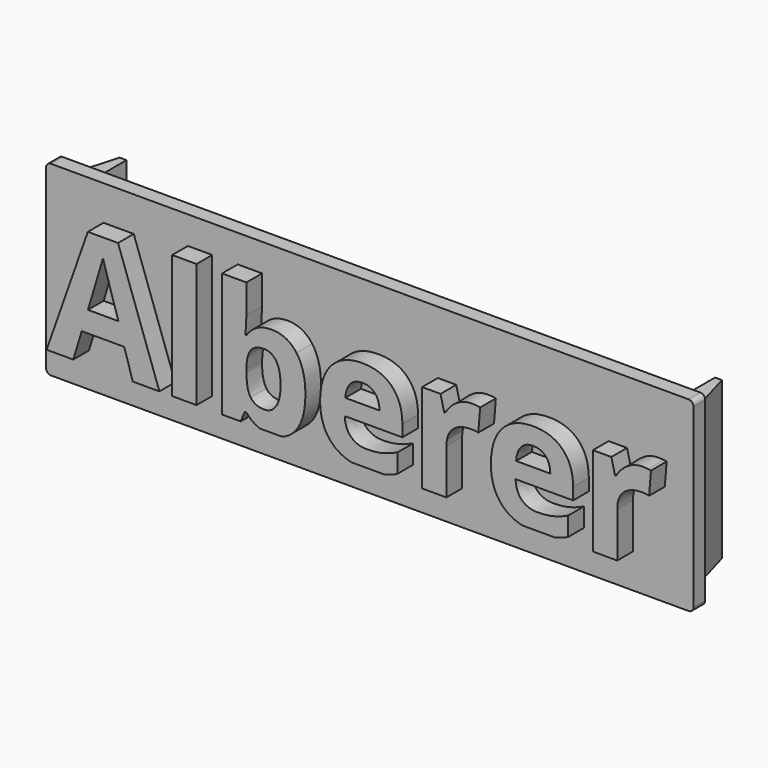
from build123d import *

# Parameters (mm, degrees)
F0_W     = 2.6041666667
F0_H     = 12
F0_W_2   = 2.4817708333
F0_W_3   = 1.2
F0_H_2   = 2
F0_H_3   = 1.5
F0_W_4   = 0.1463541667
F0_H_4   = 0.6640625
F0_W_5   = 0.5
F1_DEPTH = 1.5
F2_DEPTH = 3.5
F3_DEPTH = 5
F4_DEPTH = 1.5
F5_SIZE2 = 0.99999
F5_SIZE  = 3.49999
F6_SIZE2 = 3.49999
F6_SIZE  = 0.99999
F7_R     = 0.5


# Not quite as in the source:
# - a fillet or chamfer is up to 0.001 mm smaller than in the source, because OpenCascade refuses the exact size
# - a feature names something its author has since deleted; it is built from what else it names


with BuildPart() as f1:
    # F0 (on Front) → F1 (new body)
    with BuildSketch(Plane.XZ):
        with BuildLine():
            Line((30, 3.2387564007), (30, 6))
            Line((30, 6), (-10.9765625, 6))
            Line((-10.9765625, 6), (-10.9765625, 3.7161458333))
            add(Edge.make_bspline(
                [(-10.9765625, 3.7161458333), (-10.9765625, 3.15625), (-11.0729166667, 1.9192708333)],
                knots=[0, 0, 0, 1, 1, 1], degree=2))
            Line((-11.0729166667, 1.9192708333), (-10.9765625, 1.9192708333))
            add(Edge.make_bspline(
                [(-10.9765625, 1.9192708333), (-10.1041666667, 3.2682291667), (-8.3958333333, 3.2682291667)],
                knots=[0, 0, 0, 1, 1, 1], degree=2))
            add(Edge.make_bspline(
                [(-8.3958333333, 3.2682291667), (-6.7838541667, 3.2682291667), (-5.8723958333, 2.01171875)],
                knots=[0, 0, 0, 1, 1, 1], degree=2))
            add(Edge.make_bspline(
                [(-5.8723958333, 2.01171875), (-4.9609375, 0.7552083333), (-4.9609375, -1.4348958333)],
                knots=[0, 0, 0, 1, 1, 1], degree=2))
            add(Edge.make_bspline(
                [(-4.9609375, -1.4348958333), (-4.9609375, -3.6875), (-5.9010416667, -4.92578125)],
                knots=[0, 0, 0, 1, 1, 1], degree=2))
            add(Edge.make_bspline(
                [(-5.9010416667, -4.92578125), (-6.4989529355, -5.7133347356), (-7.3717996948, -6)],
                knots=[0, 0, 0, 0.6360053385, 0.6360053385, 0.6360053385], degree=2))
            Line((-7.3717996948, -6), (-0.2790829179, -6))
            add(Edge.make_bspline(
                [(-0.2790829179, -6), (-1.4444034881, -5.7178599903), (-2.2265625, -4.9505208333)],
                knots=[0.3676861883, 0.3676861883, 0.3676861883, 1, 1, 1], degree=2))
            add(Edge.make_bspline(
                [(-2.2265625, -4.9505208333), (-3.4635416667, -3.7369791667), (-3.4635416667, -1.515625)],
                knots=[0, 0, 0, 1, 1, 1], degree=2))
            add(Edge.make_bspline(
                [(-3.4635416667, -1.515625), (-3.4635416667, 0.7708333333), (-2.3203125, 2.01953125)],
                knots=[0, 0, 0, 1, 1, 1], degree=2))
            add(Edge.make_bspline(
                [(-2.3203125, 2.01953125), (-1.1770833333, 3.2682291667), (0.8411458333, 3.2682291667)],
                knots=[0, 0, 0, 1, 1, 1], degree=2))
            add(Edge.make_bspline(
                [(0.8411458333, 3.2682291667), (2.7682291667, 3.2682291667), (3.8424479167, 2.1705729167)],
                knots=[0, 0, 0, 1, 1, 1], degree=2))
            add(Edge.make_bspline(
                [(3.8424479167, 2.1705729167), (4.9166666667, 1.0729166667), (4.9166666667, -0.8645833333)],
                knots=[0, 0, 0, 1, 1, 1], degree=2))
            Line((4.9166666667, -0.8645833333), (4.9166666667, -2.0703125))
            Line((4.9166666667, -2.0703125), (-0.9505208333, -2.0703125))
            add(Edge.make_bspline(
                [(-0.9505208333, -2.0703125), (-0.9088541667, -3.1276041667), (-0.3229166667, -3.7213541667)],
                knots=[0, 0, 0, 1, 1, 1], degree=2))
            add(Edge.make_bspline(
                [(-0.3229166667, -3.7213541667), (0.2630208333, -4.3151041667), (1.3203125, -4.3151041667)],
                knots=[0, 0, 0, 1, 1, 1], degree=2))
            add(Edge.make_bspline(
                [(1.3203125, -4.3151041667), (2.1432291667, -4.3151041667), (2.875, -4.14453125)],
                knots=[0, 0, 0, 1, 1, 1], degree=2))
            add(Edge.make_bspline(
                [(2.875, -4.14453125), (3.6067708333, -3.9739583333), (4.4036458333, -3.5989583333)],
                knots=[0, 0, 0, 1, 1, 1], degree=2))
            Line((4.4036458333, -3.5989583333), (4.4036458333, -5.5208333333))
            add(Edge.make_bspline(
                [(4.4036458333, -5.5208333333), (3.7631867419, -5.841062879), (3.0370410498, -6)],
                knots=[0, 0, 0, 0.9837451644, 0.9837451644, 0.9837451644], degree=2))
            Line((3.0370410498, -6), (6.9348958333, -6))
            Line((6.9348958333, -6), (6.9348958333, 3.0989583333))
            Line((6.9348958333, 3.0989583333), (8.8151041667, 3.0989583333))
            Line((8.8151041667, 3.0989583333), (9.1822916667, 1.5677083333))
            Line((9.1822916667, 1.5677083333), (9.3020833333, 1.5677083333))
            add(Edge.make_bspline(
                [(9.3020833333, 1.5677083333), (9.7265625, 2.3333333333), (10.4466145833, 2.80078125)],
                knots=[0, 0, 0, 1, 1, 1], degree=2))
            add(Edge.make_bspline(
                [(10.4466145833, 2.80078125), (11.1666666667, 3.2682291667), (12.0130208333, 3.2682291667)],
                knots=[0, 0, 0, 1, 1, 1], degree=2))
            add(Edge.make_bspline(
                [(12.0130208333, 3.2682291667), (12.5182291667, 3.2682291667), (12.8515625, 3.1953125)],
                knots=[0, 0, 0, 1, 1, 1], degree=2))
            Line((12.8515625, 3.1953125), (12.6640625, 0.8697916667))
            add(Edge.make_bspline(
                [(12.6640625, 0.8697916667), (12.3619791667, 0.9505208333), (11.9322916667, 0.9505208333)],
                knots=[0, 0, 0, 1, 1, 1], degree=2))
            add(Edge.make_bspline(
                [(11.9322916667, 0.9505208333), (10.7447916667, 0.9505208333), (10.0807291667, 0.33984375)],
                knots=[0, 0, 0, 1, 1, 1], degree=2))
            add(Edge.make_bspline(
                [(10.0807291667, 0.33984375), (9.4166666667, -0.2708333333), (9.4166666667, -1.3697916667)],
                knots=[0, 0, 0, 1, 1, 1], degree=2))
            Line((9.4166666667, -1.3697916667), (9.4166666667, -6))
            Line((9.4166666667, -6), (17.1349795821, -6))
            add(Edge.make_bspline(
                [(17.1349795821, -6), (15.9696590119, -5.7178599903), (15.1875, -4.9505208333)],
                knots=[0.3676861883, 0.3676861883, 0.3676861883, 1, 1, 1], degree=2))
            add(Edge.make_bspline(
                [(15.1875, -4.9505208333), (13.9505208333, -3.7369791667), (13.9505208333, -1.515625)],
                knots=[0, 0, 0, 1, 1, 1], degree=2))
            add(Edge.make_bspline(
                [(13.9505208333, -1.515625), (13.9505208333, 0.7708333333), (15.09375, 2.01953125)],
                knots=[0, 0, 0, 1, 1, 1], degree=2))
            add(Edge.make_bspline(
                [(15.09375, 2.01953125), (16.2369791667, 3.2682291667), (18.2552083333, 3.2682291667)],
                knots=[0, 0, 0, 1, 1, 1], degree=2))
            add(Edge.make_bspline(
                [(18.2552083333, 3.2682291667), (20.1822916667, 3.2682291667), (21.2565104167, 2.1705729167)],
                knots=[0, 0, 0, 1, 1, 1], degree=2))
            add(Edge.make_bspline(
                [(21.2565104167, 2.1705729167), (22.3307291667, 1.0729166667), (22.3307291667, -0.8645833333)],
                knots=[0, 0, 0, 1, 1, 1], degree=2))
            Line((22.3307291667, -0.8645833333), (22.3307291667, -2.0703125))
            Line((22.3307291667, -2.0703125), (16.4635416667, -2.0703125))
            add(Edge.make_bspline(
                [(16.4635416667, -2.0703125), (16.5052083333, -3.1276041667), (17.0911458333, -3.7213541667)],
                knots=[0, 0, 0, 1, 1, 1], degree=2))
            add(Edge.make_bspline(
                [(17.0911458333, -3.7213541667), (17.6770833333, -4.3151041667), (18.734375, -4.3151041667)],
                knots=[0, 0, 0, 1, 1, 1], degree=2))
            add(Edge.make_bspline(
                [(18.734375, -4.3151041667), (19.5572916667, -4.3151041667), (20.2890625, -4.14453125)],
                knots=[0, 0, 0, 1, 1, 1], degree=2))
            add(Edge.make_bspline(
                [(20.2890625, -4.14453125), (21.0208333333, -3.9739583333), (21.8177083333, -3.5989583333)],
                knots=[0, 0, 0, 1, 1, 1], degree=2))
            Line((21.8177083333, -3.5989583333), (21.8177083333, -5.5208333333))
            add(Edge.make_bspline(
                [(21.8177083333, -5.5208333333), (21.1772492419, -5.841062879), (20.4511035498, -6)],
                knots=[0, 0, 0, 0.9837451644, 0.9837451644, 0.9837451644], degree=2))
            Line((20.4511035498, -6), (24.3489583333, -6))
            Line((24.3489583333, -6), (24.3489583333, 3.0989583333))
            Line((24.3489583333, 3.0989583333), (26.2291666667, 3.0989583333))
            Line((26.2291666667, 3.0989583333), (26.5963541667, 1.5677083333))
            Line((26.5963541667, 1.5677083333), (26.7161458333, 1.5677083333))
            add(Edge.make_bspline(
                [(26.7161458333, 1.5677083333), (27.140625, 2.3333333333), (27.8606770833, 2.80078125)],
                knots=[0, 0, 0, 1, 1, 1], degree=2))
            add(Edge.make_bspline(
                [(27.8606770833, 2.80078125), (28.5807291667, 3.2682291667), (29.4270833333, 3.2682291667)],
                knots=[0, 0, 0, 1, 1, 1], degree=2))
            add(Edge.make_bspline(
                [(29.4270833333, 3.2682291667), (29.7482774266, 3.2682291667), (30, 3.2387564007)],
                knots=[0, 0, 0, 0.6357656279, 0.6357656279, 0.6357656279], degree=2))
        make_face()
        with BuildLine():
            Line((-30, -9.5), (30, -9.5))
            Line((30, -9.5), (30, -8))
            Line((30, -8), (30, -6))
            Line((30, -6), (26.8307291667, -6))
            Line((26.8307291667, -6), (24.3489583333, -6))
            Line((24.3489583333, -6), (20.4511035498, -6))
            add(Edge.make_bspline(
                [(20.4511035498, -6), (20.4391051388, -6.002626185), (20.4270833333, -6.0052083333)],
                knots=[0.9837451644, 0.9837451644, 0.9837451644, 1, 1, 1], degree=2))
            add(Edge.make_bspline(
                [(20.4270833333, -6.0052083333), (19.6875, -6.1640625), (18.6197916667, -6.1640625)],
                knots=[0, 0, 0, 1, 1, 1], degree=2))
            add(Edge.make_bspline(
                [(18.6197916667, -6.1640625), (17.8126055815, -6.1640625), (17.1349795821, -6)],
                knots=[0, 0, 0, 0.3676861883, 0.3676861883, 0.3676861883], degree=2))
            Line((17.1349795821, -6), (9.4166666667, -6))
            Line((9.4166666667, -6), (6.9348958333, -6))
            Line((6.9348958333, -6), (3.0370410498, -6))
            add(Edge.make_bspline(
                [(3.0370410498, -6), (3.0250426388, -6.002626185), (3.0130208333, -6.0052083333)],
                knots=[0.9837451644, 0.9837451644, 0.9837451644, 1, 1, 1], degree=2))
            add(Edge.make_bspline(
                [(3.0130208333, -6.0052083333), (2.2734375, -6.1640625), (1.2057291667, -6.1640625)],
                knots=[0, 0, 0, 1, 1, 1], degree=2))
            add(Edge.make_bspline(
                [(1.2057291667, -6.1640625), (0.3985430815, -6.1640625), (-0.2790829179, -6)],
                knots=[0, 0, 0, 0.3676861883, 0.3676861883, 0.3676861883], degree=2))
            Line((-0.2790829179, -6), (-7.3717996948, -6))
            add(Edge.make_bspline(
                [(-7.3717996948, -6), (-7.8713419807, -6.1640625), (-8.4609375, -6.1640625)],
                knots=[0.6360053385, 0.6360053385, 0.6360053385, 1, 1, 1], degree=2))
            add(Edge.make_bspline(
                [(-8.4609375, -6.1640625), (-9.0631725128, -6.1640625), (-9.567777492, -6)],
                knots=[0, 0, 0, 0.3754192288, 0.3754192288, 0.3754192288], degree=2))
            Line((-9.567777492, -6), (-11.5625, -6))
            Line((-11.5625, -6), (-13.4583333333, -6))
            Line((-13.4583333333, -6), (-16.0625, -6))
            Line((-16.0625, -6), (-18.5442708333, -6))
            Line((-18.5442708333, -6), (-19.8463541667, -6))
            Line((-19.8463541667, -6), (-22.5651041667, -6))
            Line((-22.5651041667, -6), (-28.6276041667, -6))
            Line((-28.6276041667, -6), (-30, -6))
            Line((-30, -6), (-30, -8))
            Line((-30, -8), (-30, -9.5))
        make_face()
        Polygon((30, 8), (30, 9.5), (-30, 9.5), (-30, 8), (-30, 6), (-18.5442708333, 6), (-18.5442708333, 6.6640625), (-16.0625, 6.6640625), (-16.0625, 6), (-13.4583333333, 6), (-13.4583333333, 6.6640625), (-10.9765625, 6.6640625), (-10.9765625, 6), (30, 6), align=None)
        with BuildLine():
            Line((-10.9765625, 3.7161458333), (-10.9765625, 6))
            Line((-10.9765625, 6), (-13.4583333333, 6))
            Line((-13.4583333333, 6), (-13.4583333333, -6))
            Line((-13.4583333333, -6), (-11.5625, -6))
            Line((-11.5625, -6), (-11.1458333333, -5))
            Line((-11.1458333333, -5), (-10.9765625, -5))
            add(Edge.make_bspline(
                [(-9.567777492, -6), (-10.4072831512, -5.727051054), (-10.9765625, -5)],
                knots=[0.3754192288, 0.3754192288, 0.3754192288, 1, 1, 1], degree=2))
            Line((-9.567777492, -6), (-7.3717996948, -6))
            add(Edge.make_bspline(
                [(-5.9010416667, -4.92578125), (-6.4989529355, -5.7133347356), (-7.3717996948, -6)],
                knots=[0, 0, 0, 0.6360053385, 0.6360053385, 0.6360053385], degree=2))
            add(Edge.make_bspline(
                [(-4.9609375, -1.4348958333), (-4.9609375, -3.6875), (-5.9010416667, -4.92578125)],
                knots=[0, 0, 0, 1, 1, 1], degree=2))
            add(Edge.make_bspline(
                [(-5.8723958333, 2.01171875), (-4.9609375, 0.7552083333), (-4.9609375, -1.4348958333)],
                knots=[0, 0, 0, 1, 1, 1], degree=2))
            add(Edge.make_bspline(
                [(-8.3958333333, 3.2682291667), (-6.7838541667, 3.2682291667), (-5.8723958333, 2.01171875)],
                knots=[0, 0, 0, 1, 1, 1], degree=2))
            add(Edge.make_bspline(
                [(-10.9765625, 1.9192708333), (-10.1041666667, 3.2682291667), (-8.3958333333, 3.2682291667)],
                knots=[0, 0, 0, 1, 1, 1], degree=2))
            Line((-10.9765625, 1.9192708333), (-11.0729166667, 1.9192708333))
            add(Edge.make_bspline(
                [(-10.9765625, 3.7161458333), (-10.9765625, 3.15625), (-11.0729166667, 1.9192708333)],
                knots=[0, 0, 0, 1, 1, 1], degree=2))
        make_face()
        with BuildLine():
            add(Edge.make_bspline(
                [(-9.1927083333, 1.2838541667), (-10.1145833333, 1.2838541667), (-10.5377604167, 0.71875)],
                knots=[0, 0, 0, 1, 1, 1], degree=2))
            add(Edge.make_bspline(
                [(-7.9479166667, 0.6119791667), (-8.4036458333, 1.2838541667), (-9.1927083333, 1.2838541667)],
                knots=[0, 0, 0, 1, 1, 1], degree=2))
            add(Edge.make_bspline(
                [(-7.4921875, -1.4010416667), (-7.4921875, -0.0598958333), (-7.9479166667, 0.6119791667)],
                knots=[0, 0, 0, 1, 1, 1], degree=2))
            add(Edge.make_bspline(
                [(-7.9440104167, -3.44921875), (-7.4921875, -2.7447916667), (-7.4921875, -1.4010416667)],
                knots=[0, 0, 0, 1, 1, 1], degree=2))
            add(Edge.make_bspline(
                [(-9.1614583333, -4.1536458333), (-8.3958333333, -4.1536458333), (-7.9440104167, -3.44921875)],
                knots=[0, 0, 0, 1, 1, 1], degree=2))
            add(Edge.make_bspline(
                [(-10.5403645833, -3.5182291667), (-10.1041666667, -4.1536458333), (-9.1614583333, -4.1536458333)],
                knots=[0, 0, 0, 1, 1, 1], degree=2))
            add(Edge.make_bspline(
                [(-10.9765625, -1.4192708333), (-10.9765625, -2.8828125), (-10.5403645833, -3.5182291667)],
                knots=[0, 0, 0, 1, 1, 1], degree=2))
            Line((-10.9765625, -1.4192708333), (-10.9765625, -1.1484375))
            add(Edge.make_bspline(
                [(-10.5377604167, 0.71875), (-10.9609375, 0.1536458333), (-10.9765625, -1.1484375)],
                knots=[0, 0, 0, 1, 1, 1], degree=2))
        make_face(mode=Mode.SUBTRACT)
        Polygon((-30, -2.170444565), (-30, -6), (-28.6276041667, -6), (-27.765625, -3.1666666667), (-23.4270833333, -3.1666666667), (-22.5651041667, -6), (-19.8463541667, -6), (-24.0625, 5.9479166667), (-27.1458333333, 5.9479166667), align=None)
        with BuildLine():
            add(Edge.make_bspline(
                [(-24.03125, -1.0520833333), (-25.2265625, 2.796875), (-25.3776041667, 3.3020833333)],
                knots=[0, 0, 0, 1, 1, 1], degree=2))
            Line((-24.03125, -1.0520833333), (-27.1302083333, -1.0520833333))
            add(Edge.make_bspline(
                [(-25.59375, 4.0989583333), (-25.8619791667, 3.0572916667), (-27.1302083333, -1.0520833333)],
                knots=[0, 0, 0, 1, 1, 1], degree=2))
            add(Edge.make_bspline(
                [(-25.3776041667, 3.3020833333), (-25.5286458333, 3.8072916667), (-25.59375, 4.0989583333)],
                knots=[0, 0, 0, 1, 1, 1], degree=2))
        make_face(mode=Mode.SUBTRACT)
        with BuildLine():
            Line((-0.2790829179, -6), (3.0370410498, -6))
            add(Edge.make_bspline(
                [(4.4036458333, -5.5208333333), (3.7631867419, -5.841062879), (3.0370410498, -6)],
                knots=[0, 0, 0, 0.9837451644, 0.9837451644, 0.9837451644], degree=2))
            Line((4.4036458333, -5.5208333333), (4.4036458333, -3.5989583333))
            add(Edge.make_bspline(
                [(2.875, -4.14453125), (3.6067708333, -3.9739583333), (4.4036458333, -3.5989583333)],
                knots=[0, 0, 0, 1, 1, 1], degree=2))
            add(Edge.make_bspline(
                [(1.3203125, -4.3151041667), (2.1432291667, -4.3151041667), (2.875, -4.14453125)],
                knots=[0, 0, 0, 1, 1, 1], degree=2))
            add(Edge.make_bspline(
                [(-0.3229166667, -3.7213541667), (0.2630208333, -4.3151041667), (1.3203125, -4.3151041667)],
                knots=[0, 0, 0, 1, 1, 1], degree=2))
            add(Edge.make_bspline(
                [(-0.9505208333, -2.0703125), (-0.9088541667, -3.1276041667), (-0.3229166667, -3.7213541667)],
                knots=[0, 0, 0, 1, 1, 1], degree=2))
            Line((-0.9505208333, -2.0703125), (4.9166666667, -2.0703125))
            Line((4.9166666667, -2.0703125), (4.9166666667, -0.8645833333))
            add(Edge.make_bspline(
                [(3.8424479167, 2.1705729167), (4.9166666667, 1.0729166667), (4.9166666667, -0.8645833333)],
                knots=[0, 0, 0, 1, 1, 1], degree=2))
            add(Edge.make_bspline(
                [(0.8411458333, 3.2682291667), (2.7682291667, 3.2682291667), (3.8424479167, 2.1705729167)],
                knots=[0, 0, 0, 1, 1, 1], degree=2))
            add(Edge.make_bspline(
                [(-2.3203125, 2.01953125), (-1.1770833333, 3.2682291667), (0.8411458333, 3.2682291667)],
                knots=[0, 0, 0, 1, 1, 1], degree=2))
            add(Edge.make_bspline(
                [(-3.4635416667, -1.515625), (-3.4635416667, 0.7708333333), (-2.3203125, 2.01953125)],
                knots=[0, 0, 0, 1, 1, 1], degree=2))
            add(Edge.make_bspline(
                [(-2.2265625, -4.9505208333), (-3.4635416667, -3.7369791667), (-3.4635416667, -1.515625)],
                knots=[0, 0, 0, 1, 1, 1], degree=2))
            add(Edge.make_bspline(
                [(-0.2790829179, -6), (-1.4444034881, -5.7178599903), (-2.2265625, -4.9505208333)],
                knots=[0.3676861883, 0.3676861883, 0.3676861883, 1, 1, 1], degree=2))
        make_face()
        with BuildLine():
            add(Edge.make_bspline(
                [(0.8567708333, 1.5026041667), (0.0677083333, 1.5026041667), (-0.3802083333, 1.0026041667)],
                knots=[0, 0, 0, 1, 1, 1], degree=2))
            add(Edge.make_bspline(
                [(2.109375, 1.0026041667), (1.6458333333, 1.5026041667), (0.8567708333, 1.5026041667)],
                knots=[0, 0, 0, 1, 1, 1], degree=2))
            add(Edge.make_bspline(
                [(2.5911458333, -0.4166666667), (2.5729166667, 0.5026041667), (2.109375, 1.0026041667)],
                knots=[0, 0, 0, 1, 1, 1], degree=2))
            Line((2.5911458333, -0.4166666667), (-0.8932291667, -0.4166666667))
            add(Edge.make_bspline(
                [(-0.3802083333, 1.0026041667), (-0.828125, 0.5026041667), (-0.8932291667, -0.4166666667)],
                knots=[0, 0, 0, 1, 1, 1], degree=2))
        make_face(mode=Mode.SUBTRACT)
        with BuildLine():
            Line((17.1349795821, -6), (20.4511035498, -6))
            add(Edge.make_bspline(
                [(21.8177083333, -5.5208333333), (21.1772492419, -5.841062879), (20.4511035498, -6)],
                knots=[0, 0, 0, 0.9837451644, 0.9837451644, 0.9837451644], degree=2))
            Line((21.8177083333, -5.5208333333), (21.8177083333, -3.5989583333))
            add(Edge.make_bspline(
                [(20.2890625, -4.14453125), (21.0208333333, -3.9739583333), (21.8177083333, -3.5989583333)],
                knots=[0, 0, 0, 1, 1, 1], degree=2))
            add(Edge.make_bspline(
                [(18.734375, -4.3151041667), (19.5572916667, -4.3151041667), (20.2890625, -4.14453125)],
                knots=[0, 0, 0, 1, 1, 1], degree=2))
            add(Edge.make_bspline(
                [(17.0911458333, -3.7213541667), (17.6770833333, -4.3151041667), (18.734375, -4.3151041667)],
                knots=[0, 0, 0, 1, 1, 1], degree=2))
            add(Edge.make_bspline(
                [(16.4635416667, -2.0703125), (16.5052083333, -3.1276041667), (17.0911458333, -3.7213541667)],
                knots=[0, 0, 0, 1, 1, 1], degree=2))
            Line((16.4635416667, -2.0703125), (22.3307291667, -2.0703125))
            Line((22.3307291667, -2.0703125), (22.3307291667, -0.8645833333))
            add(Edge.make_bspline(
                [(21.2565104167, 2.1705729167), (22.3307291667, 1.0729166667), (22.3307291667, -0.8645833333)],
                knots=[0, 0, 0, 1, 1, 1], degree=2))
            add(Edge.make_bspline(
                [(18.2552083333, 3.2682291667), (20.1822916667, 3.2682291667), (21.2565104167, 2.1705729167)],
                knots=[0, 0, 0, 1, 1, 1], degree=2))
            add(Edge.make_bspline(
                [(15.09375, 2.01953125), (16.2369791667, 3.2682291667), (18.2552083333, 3.2682291667)],
                knots=[0, 0, 0, 1, 1, 1], degree=2))
            add(Edge.make_bspline(
                [(13.9505208333, -1.515625), (13.9505208333, 0.7708333333), (15.09375, 2.01953125)],
                knots=[0, 0, 0, 1, 1, 1], degree=2))
            add(Edge.make_bspline(
                [(15.1875, -4.9505208333), (13.9505208333, -3.7369791667), (13.9505208333, -1.515625)],
                knots=[0, 0, 0, 1, 1, 1], degree=2))
            add(Edge.make_bspline(
                [(17.1349795821, -6), (15.9696590119, -5.7178599903), (15.1875, -4.9505208333)],
                knots=[0.3676861883, 0.3676861883, 0.3676861883, 1, 1, 1], degree=2))
        make_face()
        with BuildLine():
            add(Edge.make_bspline(
                [(18.2708333333, 1.5026041667), (17.4817708333, 1.5026041667), (17.0338541667, 1.0026041667)],
                knots=[0, 0, 0, 1, 1, 1], degree=2))
            add(Edge.make_bspline(
                [(19.5234375, 1.0026041667), (19.0598958333, 1.5026041667), (18.2708333333, 1.5026041667)],
                knots=[0, 0, 0, 1, 1, 1], degree=2))
            add(Edge.make_bspline(
                [(20.0052083333, -0.4166666667), (19.9869791667, 0.5026041667), (19.5234375, 1.0026041667)],
                knots=[0, 0, 0, 1, 1, 1], degree=2))
            Line((20.0052083333, -0.4166666667), (16.5208333333, -0.4166666667))
            add(Edge.make_bspline(
                [(17.0338541667, 1.0026041667), (16.5859375, 0.5026041667), (16.5208333333, -0.4166666667)],
                knots=[0, 0, 0, 1, 1, 1], degree=2))
        make_face(mode=Mode.SUBTRACT)
        Polygon((-30, 6), (-30, -2.170444565), (-27.1458333333, 5.9479166667), (-24.0625, 5.9479166667), (-19.8463541667, -6), (-18.5442708333, -6), (-18.5442708333, 6), align=None)
        with Locations((-14.7604166667, 0)):
            Rectangle(F0_W, F0_H)
        with Locations((-17.3033854167, 0)):
            Rectangle(F0_W_2, F0_H)
        with BuildLine():
            Line((6.9348958333, -6), (9.4166666667, -6))
            Line((9.4166666667, -6), (9.4166666667, -1.3697916667))
            add(Edge.make_bspline(
                [(10.0807291667, 0.33984375), (9.4166666667, -0.2708333333), (9.4166666667, -1.3697916667)],
                knots=[0, 0, 0, 1, 1, 1], degree=2))
            add(Edge.make_bspline(
                [(11.9322916667, 0.9505208333), (10.7447916667, 0.9505208333), (10.0807291667, 0.33984375)],
                knots=[0, 0, 0, 1, 1, 1], degree=2))
            add(Edge.make_bspline(
                [(12.6640625, 0.8697916667), (12.3619791667, 0.9505208333), (11.9322916667, 0.9505208333)],
                knots=[0, 0, 0, 1, 1, 1], degree=2))
            Line((12.6640625, 0.8697916667), (12.8515625, 3.1953125))
            add(Edge.make_bspline(
                [(12.0130208333, 3.2682291667), (12.5182291667, 3.2682291667), (12.8515625, 3.1953125)],
                knots=[0, 0, 0, 1, 1, 1], degree=2))
            add(Edge.make_bspline(
                [(10.4466145833, 2.80078125), (11.1666666667, 3.2682291667), (12.0130208333, 3.2682291667)],
                knots=[0, 0, 0, 1, 1, 1], degree=2))
            add(Edge.make_bspline(
                [(9.3020833333, 1.5677083333), (9.7265625, 2.3333333333), (10.4466145833, 2.80078125)],
                knots=[0, 0, 0, 1, 1, 1], degree=2))
            Line((9.3020833333, 1.5677083333), (9.1822916667, 1.5677083333))
            Line((9.1822916667, 1.5677083333), (8.8151041667, 3.0989583333))
            Line((8.8151041667, 3.0989583333), (6.9348958333, 3.0989583333))
            Line((6.9348958333, 3.0989583333), (6.9348958333, -6))
        make_face()
        with BuildLine():
            Line((24.3489583333, -6), (26.8307291667, -6))
            Line((26.8307291667, -6), (26.8307291667, -1.3697916667))
            add(Edge.make_bspline(
                [(27.4947916667, 0.33984375), (26.8307291667, -0.2708333333), (26.8307291667, -1.3697916667)],
                knots=[0, 0, 0, 1, 1, 1], degree=2))
            add(Edge.make_bspline(
                [(29.3463541667, 0.9505208333), (28.1588541667, 0.9505208333), (27.4947916667, 0.33984375)],
                knots=[0, 0, 0, 1, 1, 1], degree=2))
            add(Edge.make_bspline(
                [(30, 0.888848029), (29.7219184932, 0.9505208333), (29.3463541667, 0.9505208333)],
                knots=[0.1259593855, 0.1259593855, 0.1259593855, 1, 1, 1], degree=2))
            Line((30, 0.888848029), (30, 3.2387564007))
            add(Edge.make_bspline(
                [(29.4270833333, 3.2682291667), (29.7482774266, 3.2682291667), (30, 3.2387564007)],
                knots=[0, 0, 0, 0.6357656279, 0.6357656279, 0.6357656279], degree=2))
            add(Edge.make_bspline(
                [(27.8606770833, 2.80078125), (28.5807291667, 3.2682291667), (29.4270833333, 3.2682291667)],
                knots=[0, 0, 0, 1, 1, 1], degree=2))
            add(Edge.make_bspline(
                [(26.7161458333, 1.5677083333), (27.140625, 2.3333333333), (27.8606770833, 2.80078125)],
                knots=[0, 0, 0, 1, 1, 1], degree=2))
            Line((26.7161458333, 1.5677083333), (26.5963541667, 1.5677083333))
            Line((26.5963541667, 1.5677083333), (26.2291666667, 3.0989583333))
            Line((26.2291666667, 3.0989583333), (24.3489583333, 3.0989583333))
            Line((24.3489583333, 3.0989583333), (24.3489583333, -6))
        make_face()
        Polygon((31.7, -9.5), (33, -9.5), (33, 9.5), (31.7, 9.5), (31.7, 8), (31.7, -8), align=None)
        Polygon((-33, -9.5), (-31.7, -9.5), (-31.7, -8), (-31.7, 8), (-31.7, 9.5), (-33, 9.5), align=None)
        with BuildLine():
            Line((26.8307291667, -6), (30, -6))
            Line((30, -6), (30, 0.888848029))
            add(Edge.make_bspline(
                [(30, 0.888848029), (29.7219184932, 0.9505208333), (29.3463541667, 0.9505208333)],
                knots=[0.1259593855, 0.1259593855, 0.1259593855, 1, 1, 1], degree=2))
            add(Edge.make_bspline(
                [(29.3463541667, 0.9505208333), (28.1588541667, 0.9505208333), (27.4947916667, 0.33984375)],
                knots=[0, 0, 0, 1, 1, 1], degree=2))
            add(Edge.make_bspline(
                [(27.4947916667, 0.33984375), (26.8307291667, -0.2708333333), (26.8307291667, -1.3697916667)],
                knots=[0, 0, 0, 1, 1, 1], degree=2))
            Line((26.8307291667, -1.3697916667), (26.8307291667, -6))
        make_face()
        with BuildLine():
            add(Edge.make_bspline(
                [(-7.9479166667, 0.6119791667), (-8.4036458333, 1.2838541667), (-9.1927083333, 1.2838541667)],
                knots=[0, 0, 0, 1, 1, 1], degree=2))
            add(Edge.make_bspline(
                [(-9.1927083333, 1.2838541667), (-10.1145833333, 1.2838541667), (-10.5377604167, 0.71875)],
                knots=[0, 0, 0, 1, 1, 1], degree=2))
            add(Edge.make_bspline(
                [(-10.5377604167, 0.71875), (-10.9609375, 0.1536458333), (-10.9765625, -1.1484375)],
                knots=[0, 0, 0, 1, 1, 1], degree=2))
            Line((-10.9765625, -1.1484375), (-10.9765625, -1.4192708333))
            add(Edge.make_bspline(
                [(-10.9765625, -1.4192708333), (-10.9765625, -2.8828125), (-10.5403645833, -3.5182291667)],
                knots=[0, 0, 0, 1, 1, 1], degree=2))
            add(Edge.make_bspline(
                [(-10.5403645833, -3.5182291667), (-10.1041666667, -4.1536458333), (-9.1614583333, -4.1536458333)],
                knots=[0, 0, 0, 1, 1, 1], degree=2))
            add(Edge.make_bspline(
                [(-9.1614583333, -4.1536458333), (-8.3958333333, -4.1536458333), (-7.9440104167, -3.44921875)],
                knots=[0, 0, 0, 1, 1, 1], degree=2))
            add(Edge.make_bspline(
                [(-7.9440104167, -3.44921875), (-7.4921875, -2.7447916667), (-7.4921875, -1.4010416667)],
                knots=[0, 0, 0, 1, 1, 1], degree=2))
            add(Edge.make_bspline(
                [(-7.4921875, -1.4010416667), (-7.4921875, -0.0598958333), (-7.9479166667, 0.6119791667)],
                knots=[0, 0, 0, 1, 1, 1], degree=2))
        make_face()
        Polygon((-27.765625, -3.1666666667), (-28.6276041667, -6), (-22.5651041667, -6), (-23.4270833333, -3.1666666667), align=None)
        with BuildLine():
            Line((30, -6), (31.2, -6))
            Line((31.2, -6), (31.2, 6))
            Line((31.2, 6), (30, 6))
            Line((30, 6), (30, 3.2387564007))
            add(Edge.make_bspline(
                [(30, 3.2387564007), (30.1442135426, 3.2218712563), (30.265625, 3.1953125)],
                knots=[0.6357656279, 0.6357656279, 0.6357656279, 1, 1, 1], degree=2))
            Line((30.265625, 3.1953125), (30.078125, 0.8697916667))
            add(Edge.make_bspline(
                [(30.078125, 0.8697916667), (30.040074769, 0.8799602629), (30, 0.888848029)],
                knots=[0, 0, 0, 0.1259593855, 0.1259593855, 0.1259593855], degree=2))
            Line((30, 0.888848029), (30, -6))
        make_face()
        Polygon((-31.2, -5.583711769), (-30, -2.170444565), (-30, 6), (-31.2, 6), align=None)
        with BuildLine():
            Line((-27.1302083333, -1.0520833333), (-24.03125, -1.0520833333))
            add(Edge.make_bspline(
                [(-24.03125, -1.0520833333), (-25.2265625, 2.796875), (-25.3776041667, 3.3020833333)],
                knots=[0, 0, 0, 1, 1, 1], degree=2))
            add(Edge.make_bspline(
                [(-25.3776041667, 3.3020833333), (-25.5286458333, 3.8072916667), (-25.59375, 4.0989583333)],
                knots=[0, 0, 0, 1, 1, 1], degree=2))
            add(Edge.make_bspline(
                [(-25.59375, 4.0989583333), (-25.8619791667, 3.0572916667), (-27.1302083333, -1.0520833333)],
                knots=[0, 0, 0, 1, 1, 1], degree=2))
        make_face()
        Polygon((-31.7, -8), (-31.2, -8), (-31.2, -6), (-31.3463541667, -6), (-31.3463541667, 6), (-31.2, 6), (-31.2, 8), (-31.7, 8), align=None)
        Polygon((31.2, -8), (31.7, -8), (31.7, 8), (31.2, 8), (31.2, 6), (31.3463541667, 6), (31.3463541667, -6), (31.2, -6), align=None)
        with BuildLine():
            add(Edge.make_bspline(
                [(19.5234375, 1.0026041667), (19.0598958333, 1.5026041667), (18.2708333333, 1.5026041667)],
                knots=[0, 0, 0, 1, 1, 1], degree=2))
            add(Edge.make_bspline(
                [(18.2708333333, 1.5026041667), (17.4817708333, 1.5026041667), (17.0338541667, 1.0026041667)],
                knots=[0, 0, 0, 1, 1, 1], degree=2))
            add(Edge.make_bspline(
                [(17.0338541667, 1.0026041667), (16.5859375, 0.5026041667), (16.5208333333, -0.4166666667)],
                knots=[0, 0, 0, 1, 1, 1], degree=2))
            Line((16.5208333333, -0.4166666667), (20.0052083333, -0.4166666667))
            add(Edge.make_bspline(
                [(20.0052083333, -0.4166666667), (19.9869791667, 0.5026041667), (19.5234375, 1.0026041667)],
                knots=[0, 0, 0, 1, 1, 1], degree=2))
        make_face()
        with BuildLine():
            add(Edge.make_bspline(
                [(2.109375, 1.0026041667), (1.6458333333, 1.5026041667), (0.8567708333, 1.5026041667)],
                knots=[0, 0, 0, 1, 1, 1], degree=2))
            add(Edge.make_bspline(
                [(0.8567708333, 1.5026041667), (0.0677083333, 1.5026041667), (-0.3802083333, 1.0026041667)],
                knots=[0, 0, 0, 1, 1, 1], degree=2))
            add(Edge.make_bspline(
                [(-0.3802083333, 1.0026041667), (-0.828125, 0.5026041667), (-0.8932291667, -0.4166666667)],
                knots=[0, 0, 0, 1, 1, 1], degree=2))
            Line((-0.8932291667, -0.4166666667), (2.5911458333, -0.4166666667))
            add(Edge.make_bspline(
                [(2.5911458333, -0.4166666667), (2.5729166667, 0.5026041667), (2.109375, 1.0026041667)],
                knots=[0, 0, 0, 1, 1, 1], degree=2))
        make_face()
        Polygon((-31.2, -6), (-30, -6), (-30, -2.170444565), (-31.2, -5.583711769), align=None)
        with Locations((-30.6, 7)):
            Rectangle(F0_W_3, F0_H_2)
        with Locations((-30.6, -7)):
            Rectangle(F0_W_3, F0_H_2)
        with Locations((30.6, 7)):
            Rectangle(F0_W_3, F0_H_2)
        with Locations((30.6, -7)):
            Rectangle(F0_W_3, F0_H_2)
        with Locations((30.6, -8.75)):
            Rectangle(F0_W_3, F0_H_3)
        with Locations((30.6, 8.75)):
            Rectangle(F0_W_3, F0_H_3)
        with Locations((-30.6, -8.75)):
            Rectangle(F0_W_3, F0_H_3)
        with Locations((-30.6, 8.75)):
            Rectangle(F0_W_3, F0_H_3)
        with Locations((31.2731770833, 0)):
            Rectangle(F0_W_4, F0_H)
        Polygon((-31.3463541667, 6), (-31.3463541667, -6), (-31.2, -5.583711769), (-31.2, 6), align=None)
        with Locations((-17.3033854167, 6.33203125)):
            Rectangle(F0_W_2, F0_H_4)
        with Locations((-12.2174479167, 6.33203125)):
            Rectangle(F0_W_2, F0_H_4)
        with BuildLine():
            Line((-11.1458333333, -5), (-11.5625, -6))
            Line((-11.5625, -6), (-9.567777492, -6))
            add(Edge.make_bspline(
                [(-9.567777492, -6), (-10.4072831512, -5.727051054), (-10.9765625, -5)],
                knots=[0.3754192288, 0.3754192288, 0.3754192288, 1, 1, 1], degree=2))
            Line((-10.9765625, -5), (-11.1458333333, -5))
        make_face()
        with Locations((31.45, -8.75)):
            Rectangle(F0_W_5, F0_H_3)
        with Locations((31.45, 8.75)):
            Rectangle(F0_W_5, F0_H_3)
        with Locations((-31.45, -8.75)):
            Rectangle(F0_W_5, F0_H_3)
        with Locations((-31.45, 8.75)):
            Rectangle(F0_W_5, F0_H_3)
        with BuildLine():
            Line((30, 3.2387564007), (30, 0.888848029))
            add(Edge.make_bspline(
                [(30.078125, 0.8697916667), (30.040074769, 0.8799602629), (30, 0.888848029)],
                knots=[0, 0, 0, 0.1259593855, 0.1259593855, 0.1259593855], degree=2))
            Line((30.078125, 0.8697916667), (30.265625, 3.1953125))
            add(Edge.make_bspline(
                [(30, 3.2387564007), (30.1442135426, 3.2218712563), (30.265625, 3.1953125)],
                knots=[0.6357656279, 0.6357656279, 0.6357656279, 1, 1, 1], degree=2))
        make_face()
        with BuildLine():
            add(Edge.make_bspline(
                [(20.4511035498, -6), (20.4391051388, -6.002626185), (20.4270833333, -6.0052083333)],
                knots=[0.9837451644, 0.9837451644, 0.9837451644, 1, 1, 1], degree=2))
            Line((20.4511035498, -6), (17.1349795821, -6))
            add(Edge.make_bspline(
                [(18.6197916667, -6.1640625), (17.8126055815, -6.1640625), (17.1349795821, -6)],
                knots=[0, 0, 0, 0.3676861883, 0.3676861883, 0.3676861883], degree=2))
            add(Edge.make_bspline(
                [(20.4270833333, -6.0052083333), (19.6875, -6.1640625), (18.6197916667, -6.1640625)],
                knots=[0, 0, 0, 1, 1, 1], degree=2))
        make_face()
        with BuildLine():
            add(Edge.make_bspline(
                [(3.0370410498, -6), (3.0250426388, -6.002626185), (3.0130208333, -6.0052083333)],
                knots=[0.9837451644, 0.9837451644, 0.9837451644, 1, 1, 1], degree=2))
            Line((3.0370410498, -6), (-0.2790829179, -6))
            add(Edge.make_bspline(
                [(1.2057291667, -6.1640625), (0.3985430815, -6.1640625), (-0.2790829179, -6)],
                knots=[0, 0, 0, 0.3676861883, 0.3676861883, 0.3676861883], degree=2))
            add(Edge.make_bspline(
                [(3.0130208333, -6.0052083333), (2.2734375, -6.1640625), (1.2057291667, -6.1640625)],
                knots=[0, 0, 0, 1, 1, 1], degree=2))
        make_face()
        with BuildLine():
            Line((-7.3717996948, -6), (-9.567777492, -6))
            add(Edge.make_bspline(
                [(-8.4609375, -6.1640625), (-9.0631725128, -6.1640625), (-9.567777492, -6)],
                knots=[0, 0, 0, 0.3754192288, 0.3754192288, 0.3754192288], degree=2))
            add(Edge.make_bspline(
                [(-7.3717996948, -6), (-7.8713419807, -6.1640625), (-8.4609375, -6.1640625)],
                knots=[0.6360053385, 0.6360053385, 0.6360053385, 1, 1, 1], degree=2))
        make_face()
        Polygon((-31.3463541667, -6), (-31.2, -6), (-31.2, -5.583711769), align=None)
    extrude(amount=F1_DEPTH)

    # F0 (on Front) → F2 (join)
    with BuildSketch(Plane.XZ):
        with BuildLine():
            Line((24.3489583333, -6), (26.8307291667, -6))
            Line((26.8307291667, -6), (26.8307291667, -1.3697916667))
            add(Edge.make_bspline(
                [(27.4947916667, 0.33984375), (26.8307291667, -0.2708333333), (26.8307291667, -1.3697916667)],
                knots=[0, 0, 0, 1, 1, 1], degree=2))
            add(Edge.make_bspline(
                [(29.3463541667, 0.9505208333), (28.1588541667, 0.9505208333), (27.4947916667, 0.33984375)],
                knots=[0, 0, 0, 1, 1, 1], degree=2))
            add(Edge.make_bspline(
                [(30, 0.888848029), (29.7219184932, 0.9505208333), (29.3463541667, 0.9505208333)],
                knots=[0.1259593855, 0.1259593855, 0.1259593855, 1, 1, 1], degree=2))
            Line((30, 0.888848029), (30, 3.2387564007))
            add(Edge.make_bspline(
                [(29.4270833333, 3.2682291667), (29.7482774266, 3.2682291667), (30, 3.2387564007)],
                knots=[0, 0, 0, 0.6357656279, 0.6357656279, 0.6357656279], degree=2))
            add(Edge.make_bspline(
                [(27.8606770833, 2.80078125), (28.5807291667, 3.2682291667), (29.4270833333, 3.2682291667)],
                knots=[0, 0, 0, 1, 1, 1], degree=2))
            add(Edge.make_bspline(
                [(26.7161458333, 1.5677083333), (27.140625, 2.3333333333), (27.8606770833, 2.80078125)],
                knots=[0, 0, 0, 1, 1, 1], degree=2))
            Line((26.7161458333, 1.5677083333), (26.5963541667, 1.5677083333))
            Line((26.5963541667, 1.5677083333), (26.2291666667, 3.0989583333))
            Line((26.2291666667, 3.0989583333), (24.3489583333, 3.0989583333))
            Line((24.3489583333, 3.0989583333), (24.3489583333, -6))
        make_face()
        with BuildLine():
            Line((30, 3.2387564007), (30, 0.888848029))
            add(Edge.make_bspline(
                [(30.078125, 0.8697916667), (30.040074769, 0.8799602629), (30, 0.888848029)],
                knots=[0, 0, 0, 0.1259593855, 0.1259593855, 0.1259593855], degree=2))
            Line((30.078125, 0.8697916667), (30.265625, 3.1953125))
            add(Edge.make_bspline(
                [(30, 3.2387564007), (30.1442135426, 3.2218712563), (30.265625, 3.1953125)],
                knots=[0.6357656279, 0.6357656279, 0.6357656279, 1, 1, 1], degree=2))
        make_face()
        with BuildLine():
            Line((17.1349795821, -6), (20.4511035498, -6))
            add(Edge.make_bspline(
                [(21.8177083333, -5.5208333333), (21.1772492419, -5.841062879), (20.4511035498, -6)],
                knots=[0, 0, 0, 0.9837451644, 0.9837451644, 0.9837451644], degree=2))
            Line((21.8177083333, -5.5208333333), (21.8177083333, -3.5989583333))
            add(Edge.make_bspline(
                [(20.2890625, -4.14453125), (21.0208333333, -3.9739583333), (21.8177083333, -3.5989583333)],
                knots=[0, 0, 0, 1, 1, 1], degree=2))
            add(Edge.make_bspline(
                [(18.734375, -4.3151041667), (19.5572916667, -4.3151041667), (20.2890625, -4.14453125)],
                knots=[0, 0, 0, 1, 1, 1], degree=2))
            add(Edge.make_bspline(
                [(17.0911458333, -3.7213541667), (17.6770833333, -4.3151041667), (18.734375, -4.3151041667)],
                knots=[0, 0, 0, 1, 1, 1], degree=2))
            add(Edge.make_bspline(
                [(16.4635416667, -2.0703125), (16.5052083333, -3.1276041667), (17.0911458333, -3.7213541667)],
                knots=[0, 0, 0, 1, 1, 1], degree=2))
            Line((16.4635416667, -2.0703125), (22.3307291667, -2.0703125))
            Line((22.3307291667, -2.0703125), (22.3307291667, -0.8645833333))
            add(Edge.make_bspline(
                [(21.2565104167, 2.1705729167), (22.3307291667, 1.0729166667), (22.3307291667, -0.8645833333)],
                knots=[0, 0, 0, 1, 1, 1], degree=2))
            add(Edge.make_bspline(
                [(18.2552083333, 3.2682291667), (20.1822916667, 3.2682291667), (21.2565104167, 2.1705729167)],
                knots=[0, 0, 0, 1, 1, 1], degree=2))
            add(Edge.make_bspline(
                [(15.09375, 2.01953125), (16.2369791667, 3.2682291667), (18.2552083333, 3.2682291667)],
                knots=[0, 0, 0, 1, 1, 1], degree=2))
            add(Edge.make_bspline(
                [(13.9505208333, -1.515625), (13.9505208333, 0.7708333333), (15.09375, 2.01953125)],
                knots=[0, 0, 0, 1, 1, 1], degree=2))
            add(Edge.make_bspline(
                [(15.1875, -4.9505208333), (13.9505208333, -3.7369791667), (13.9505208333, -1.515625)],
                knots=[0, 0, 0, 1, 1, 1], degree=2))
            add(Edge.make_bspline(
                [(17.1349795821, -6), (15.9696590119, -5.7178599903), (15.1875, -4.9505208333)],
                knots=[0.3676861883, 0.3676861883, 0.3676861883, 1, 1, 1], degree=2))
        make_face()
        with BuildLine():
            add(Edge.make_bspline(
                [(18.2708333333, 1.5026041667), (17.4817708333, 1.5026041667), (17.0338541667, 1.0026041667)],
                knots=[0, 0, 0, 1, 1, 1], degree=2))
            add(Edge.make_bspline(
                [(19.5234375, 1.0026041667), (19.0598958333, 1.5026041667), (18.2708333333, 1.5026041667)],
                knots=[0, 0, 0, 1, 1, 1], degree=2))
            add(Edge.make_bspline(
                [(20.0052083333, -0.4166666667), (19.9869791667, 0.5026041667), (19.5234375, 1.0026041667)],
                knots=[0, 0, 0, 1, 1, 1], degree=2))
            Line((20.0052083333, -0.4166666667), (16.5208333333, -0.4166666667))
            add(Edge.make_bspline(
                [(17.0338541667, 1.0026041667), (16.5859375, 0.5026041667), (16.5208333333, -0.4166666667)],
                knots=[0, 0, 0, 1, 1, 1], degree=2))
        make_face(mode=Mode.SUBTRACT)
        with BuildLine():
            Line((6.9348958333, -6), (9.4166666667, -6))
            Line((9.4166666667, -6), (9.4166666667, -1.3697916667))
            add(Edge.make_bspline(
                [(10.0807291667, 0.33984375), (9.4166666667, -0.2708333333), (9.4166666667, -1.3697916667)],
                knots=[0, 0, 0, 1, 1, 1], degree=2))
            add(Edge.make_bspline(
                [(11.9322916667, 0.9505208333), (10.7447916667, 0.9505208333), (10.0807291667, 0.33984375)],
                knots=[0, 0, 0, 1, 1, 1], degree=2))
            add(Edge.make_bspline(
                [(12.6640625, 0.8697916667), (12.3619791667, 0.9505208333), (11.9322916667, 0.9505208333)],
                knots=[0, 0, 0, 1, 1, 1], degree=2))
            Line((12.6640625, 0.8697916667), (12.8515625, 3.1953125))
            add(Edge.make_bspline(
                [(12.0130208333, 3.2682291667), (12.5182291667, 3.2682291667), (12.8515625, 3.1953125)],
                knots=[0, 0, 0, 1, 1, 1], degree=2))
            add(Edge.make_bspline(
                [(10.4466145833, 2.80078125), (11.1666666667, 3.2682291667), (12.0130208333, 3.2682291667)],
                knots=[0, 0, 0, 1, 1, 1], degree=2))
            add(Edge.make_bspline(
                [(9.3020833333, 1.5677083333), (9.7265625, 2.3333333333), (10.4466145833, 2.80078125)],
                knots=[0, 0, 0, 1, 1, 1], degree=2))
            Line((9.3020833333, 1.5677083333), (9.1822916667, 1.5677083333))
            Line((9.1822916667, 1.5677083333), (8.8151041667, 3.0989583333))
            Line((8.8151041667, 3.0989583333), (6.9348958333, 3.0989583333))
            Line((6.9348958333, 3.0989583333), (6.9348958333, -6))
        make_face()
        with BuildLine():
            Line((-0.2790829179, -6), (3.0370410498, -6))
            add(Edge.make_bspline(
                [(4.4036458333, -5.5208333333), (3.7631867419, -5.841062879), (3.0370410498, -6)],
                knots=[0, 0, 0, 0.9837451644, 0.9837451644, 0.9837451644], degree=2))
            Line((4.4036458333, -5.5208333333), (4.4036458333, -3.5989583333))
            add(Edge.make_bspline(
                [(2.875, -4.14453125), (3.6067708333, -3.9739583333), (4.4036458333, -3.5989583333)],
                knots=[0, 0, 0, 1, 1, 1], degree=2))
            add(Edge.make_bspline(
                [(1.3203125, -4.3151041667), (2.1432291667, -4.3151041667), (2.875, -4.14453125)],
                knots=[0, 0, 0, 1, 1, 1], degree=2))
            add(Edge.make_bspline(
                [(-0.3229166667, -3.7213541667), (0.2630208333, -4.3151041667), (1.3203125, -4.3151041667)],
                knots=[0, 0, 0, 1, 1, 1], degree=2))
            add(Edge.make_bspline(
                [(-0.9505208333, -2.0703125), (-0.9088541667, -3.1276041667), (-0.3229166667, -3.7213541667)],
                knots=[0, 0, 0, 1, 1, 1], degree=2))
            Line((-0.9505208333, -2.0703125), (4.9166666667, -2.0703125))
            Line((4.9166666667, -2.0703125), (4.9166666667, -0.8645833333))
            add(Edge.make_bspline(
                [(3.8424479167, 2.1705729167), (4.9166666667, 1.0729166667), (4.9166666667, -0.8645833333)],
                knots=[0, 0, 0, 1, 1, 1], degree=2))
            add(Edge.make_bspline(
                [(0.8411458333, 3.2682291667), (2.7682291667, 3.2682291667), (3.8424479167, 2.1705729167)],
                knots=[0, 0, 0, 1, 1, 1], degree=2))
            add(Edge.make_bspline(
                [(-2.3203125, 2.01953125), (-1.1770833333, 3.2682291667), (0.8411458333, 3.2682291667)],
                knots=[0, 0, 0, 1, 1, 1], degree=2))
            add(Edge.make_bspline(
                [(-3.4635416667, -1.515625), (-3.4635416667, 0.7708333333), (-2.3203125, 2.01953125)],
                knots=[0, 0, 0, 1, 1, 1], degree=2))
            add(Edge.make_bspline(
                [(-2.2265625, -4.9505208333), (-3.4635416667, -3.7369791667), (-3.4635416667, -1.515625)],
                knots=[0, 0, 0, 1, 1, 1], degree=2))
            add(Edge.make_bspline(
                [(-0.2790829179, -6), (-1.4444034881, -5.7178599903), (-2.2265625, -4.9505208333)],
                knots=[0.3676861883, 0.3676861883, 0.3676861883, 1, 1, 1], degree=2))
        make_face()
        with BuildLine():
            add(Edge.make_bspline(
                [(0.8567708333, 1.5026041667), (0.0677083333, 1.5026041667), (-0.3802083333, 1.0026041667)],
                knots=[0, 0, 0, 1, 1, 1], degree=2))
            add(Edge.make_bspline(
                [(2.109375, 1.0026041667), (1.6458333333, 1.5026041667), (0.8567708333, 1.5026041667)],
                knots=[0, 0, 0, 1, 1, 1], degree=2))
            add(Edge.make_bspline(
                [(2.5911458333, -0.4166666667), (2.5729166667, 0.5026041667), (2.109375, 1.0026041667)],
                knots=[0, 0, 0, 1, 1, 1], degree=2))
            Line((2.5911458333, -0.4166666667), (-0.8932291667, -0.4166666667))
            add(Edge.make_bspline(
                [(-0.3802083333, 1.0026041667), (-0.828125, 0.5026041667), (-0.8932291667, -0.4166666667)],
                knots=[0, 0, 0, 1, 1, 1], degree=2))
        make_face(mode=Mode.SUBTRACT)
        with BuildLine():
            Line((-10.9765625, 3.7161458333), (-10.9765625, 6))
            Line((-10.9765625, 6), (-13.4583333333, 6))
            Line((-13.4583333333, 6), (-13.4583333333, -6))
            Line((-13.4583333333, -6), (-11.5625, -6))
            Line((-11.5625, -6), (-11.1458333333, -5))
            Line((-11.1458333333, -5), (-10.9765625, -5))
            add(Edge.make_bspline(
                [(-9.567777492, -6), (-10.4072831512, -5.727051054), (-10.9765625, -5)],
                knots=[0.3754192288, 0.3754192288, 0.3754192288, 1, 1, 1], degree=2))
            Line((-9.567777492, -6), (-7.3717996948, -6))
            add(Edge.make_bspline(
                [(-5.9010416667, -4.92578125), (-6.4989529355, -5.7133347356), (-7.3717996948, -6)],
                knots=[0, 0, 0, 0.6360053385, 0.6360053385, 0.6360053385], degree=2))
            add(Edge.make_bspline(
                [(-4.9609375, -1.4348958333), (-4.9609375, -3.6875), (-5.9010416667, -4.92578125)],
                knots=[0, 0, 0, 1, 1, 1], degree=2))
            add(Edge.make_bspline(
                [(-5.8723958333, 2.01171875), (-4.9609375, 0.7552083333), (-4.9609375, -1.4348958333)],
                knots=[0, 0, 0, 1, 1, 1], degree=2))
            add(Edge.make_bspline(
                [(-8.3958333333, 3.2682291667), (-6.7838541667, 3.2682291667), (-5.8723958333, 2.01171875)],
                knots=[0, 0, 0, 1, 1, 1], degree=2))
            add(Edge.make_bspline(
                [(-10.9765625, 1.9192708333), (-10.1041666667, 3.2682291667), (-8.3958333333, 3.2682291667)],
                knots=[0, 0, 0, 1, 1, 1], degree=2))
            Line((-10.9765625, 1.9192708333), (-11.0729166667, 1.9192708333))
            add(Edge.make_bspline(
                [(-10.9765625, 3.7161458333), (-10.9765625, 3.15625), (-11.0729166667, 1.9192708333)],
                knots=[0, 0, 0, 1, 1, 1], degree=2))
        make_face()
        with BuildLine():
            add(Edge.make_bspline(
                [(-9.1927083333, 1.2838541667), (-10.1145833333, 1.2838541667), (-10.5377604167, 0.71875)],
                knots=[0, 0, 0, 1, 1, 1], degree=2))
            add(Edge.make_bspline(
                [(-7.9479166667, 0.6119791667), (-8.4036458333, 1.2838541667), (-9.1927083333, 1.2838541667)],
                knots=[0, 0, 0, 1, 1, 1], degree=2))
            add(Edge.make_bspline(
                [(-7.4921875, -1.4010416667), (-7.4921875, -0.0598958333), (-7.9479166667, 0.6119791667)],
                knots=[0, 0, 0, 1, 1, 1], degree=2))
            add(Edge.make_bspline(
                [(-7.9440104167, -3.44921875), (-7.4921875, -2.7447916667), (-7.4921875, -1.4010416667)],
                knots=[0, 0, 0, 1, 1, 1], degree=2))
            add(Edge.make_bspline(
                [(-9.1614583333, -4.1536458333), (-8.3958333333, -4.1536458333), (-7.9440104167, -3.44921875)],
                knots=[0, 0, 0, 1, 1, 1], degree=2))
            add(Edge.make_bspline(
                [(-10.5403645833, -3.5182291667), (-10.1041666667, -4.1536458333), (-9.1614583333, -4.1536458333)],
                knots=[0, 0, 0, 1, 1, 1], degree=2))
            add(Edge.make_bspline(
                [(-10.9765625, -1.4192708333), (-10.9765625, -2.8828125), (-10.5403645833, -3.5182291667)],
                knots=[0, 0, 0, 1, 1, 1], degree=2))
            Line((-10.9765625, -1.4192708333), (-10.9765625, -1.1484375))
            add(Edge.make_bspline(
                [(-10.5377604167, 0.71875), (-10.9609375, 0.1536458333), (-10.9765625, -1.1484375)],
                knots=[0, 0, 0, 1, 1, 1], degree=2))
        make_face(mode=Mode.SUBTRACT)
        with Locations((-12.2174479167, 6.33203125)):
            Rectangle(F0_W_2, F0_H_4)
        with Locations((-17.3033854167, 6.33203125)):
            Rectangle(F0_W_2, F0_H_4)
        with Locations((-17.3033854167, 0)):
            Rectangle(F0_W_2, F0_H)
        Polygon((-30, -2.170444565), (-30, -6), (-28.6276041667, -6), (-27.765625, -3.1666666667), (-23.4270833333, -3.1666666667), (-22.5651041667, -6), (-19.8463541667, -6), (-24.0625, 5.9479166667), (-27.1458333333, 5.9479166667), align=None)
        with BuildLine():
            add(Edge.make_bspline(
                [(-24.03125, -1.0520833333), (-25.2265625, 2.796875), (-25.3776041667, 3.3020833333)],
                knots=[0, 0, 0, 1, 1, 1], degree=2))
            Line((-24.03125, -1.0520833333), (-27.1302083333, -1.0520833333))
            add(Edge.make_bspline(
                [(-25.59375, 4.0989583333), (-25.8619791667, 3.0572916667), (-27.1302083333, -1.0520833333)],
                knots=[0, 0, 0, 1, 1, 1], degree=2))
            add(Edge.make_bspline(
                [(-25.3776041667, 3.3020833333), (-25.5286458333, 3.8072916667), (-25.59375, 4.0989583333)],
                knots=[0, 0, 0, 1, 1, 1], degree=2))
        make_face(mode=Mode.SUBTRACT)
        Polygon((-31.3463541667, -6), (-31.2, -6), (-31.2, -5.583711769), align=None)
        Polygon((-31.2, -6), (-30, -6), (-30, -2.170444565), (-31.2, -5.583711769), align=None)
    extrude(amount=F2_DEPTH)

    # F0 (on Front) → F3 (join)
    with BuildSketch(Plane.XZ):
        with Locations((-30.6, 7)):
            Rectangle(F0_W_3, F0_H_2)
        Polygon((-31.7, -8), (-31.2, -8), (-31.2, -6), (-31.3463541667, -6), (-31.3463541667, 6), (-31.2, 6), (-31.2, 8), (-31.7, 8), align=None)
        Polygon((-31.3463541667, 6), (-31.3463541667, -6), (-31.2, -5.583711769), (-31.2, 6), align=None)
        Polygon((-31.2, -5.583711769), (-30, -2.170444565), (-30, 6), (-31.2, 6), align=None)
        Polygon((-31.2, -6), (-30, -6), (-30, -2.170444565), (-31.2, -5.583711769), align=None)
        with Locations((-30.6, -7)):
            Rectangle(F0_W_3, F0_H_2)
        with Locations((30.6, 7)):
            Rectangle(F0_W_3, F0_H_2)
        Polygon((31.2, -8), (31.7, -8), (31.7, 8), (31.2, 8), (31.2, 6), (31.3463541667, 6), (31.3463541667, -6), (31.2, -6), align=None)
        with Locations((31.2731770833, 0)):
            Rectangle(F0_W_4, F0_H)
        with BuildLine():
            Line((30, -6), (31.2, -6))
            Line((31.2, -6), (31.2, 6))
            Line((31.2, 6), (30, 6))
            Line((30, 6), (30, 3.2387564007))
            add(Edge.make_bspline(
                [(30, 3.2387564007), (30.1442135426, 3.2218712563), (30.265625, 3.1953125)],
                knots=[0.6357656279, 0.6357656279, 0.6357656279, 1, 1, 1], degree=2))
            Line((30.265625, 3.1953125), (30.078125, 0.8697916667))
            add(Edge.make_bspline(
                [(30.078125, 0.8697916667), (30.040074769, 0.8799602629), (30, 0.888848029)],
                knots=[0, 0, 0, 0.1259593855, 0.1259593855, 0.1259593855], degree=2))
            Line((30, 0.888848029), (30, -6))
        make_face()
        with Locations((30.6, -7)):
            Rectangle(F0_W_3, F0_H_2)
        Polygon((-31.3463541667, -6), (-31.2, -6), (-31.2, -5.583711769), align=None)
        with BuildLine():
            Line((30, 3.2387564007), (30, 0.888848029))
            add(Edge.make_bspline(
                [(30.078125, 0.8697916667), (30.040074769, 0.8799602629), (30, 0.888848029)],
                knots=[0, 0, 0, 0.1259593855, 0.1259593855, 0.1259593855], degree=2))
            Line((30.078125, 0.8697916667), (30.265625, 3.1953125))
            add(Edge.make_bspline(
                [(30, 3.2387564007), (30.1442135426, 3.2218712563), (30.265625, 3.1953125)],
                knots=[0.6357656279, 0.6357656279, 0.6357656279, 1, 1, 1], degree=2))
        make_face()
    extrude(amount=-F3_DEPTH)

    # F0 (on Front) → F4 (cut)
    with BuildSketch(Plane.XZ):
        Polygon((31.2, -8), (31.7, -8), (31.7, 8), (31.2, 8), (31.2, 6), (31.3463541667, 6), (31.3463541667, -6), (31.2, -6), align=None)
        with Locations((31.2731770833, 0)):
            Rectangle(F0_W_4, F0_H)
        Polygon((-31.7, -8), (-31.2, -8), (-31.2, -6), (-31.3463541667, -6), (-31.3463541667, 6), (-31.2, 6), (-31.2, 8), (-31.7, 8), align=None)
        Polygon((-31.3463541667, 6), (-31.3463541667, -6), (-31.2, -5.583711769), (-31.2, 6), align=None)
        Polygon((-31.3463541667, -6), (-31.2, -6), (-31.2, -5.583711769), align=None)
    extrude(amount=-F4_DEPTH, mode=Mode.SUBTRACT)

    # F5 (size 3.5 and 1 in the source; OpenCascade refuses exactly that, so slightly less here)
    f5_edges = [f1.edges().sort_by_distance(p)[0] for p in [
        (-31.7, 5, 0),
    ]]
    f5_side = f1.faces().sort_by_distance((-31.7, 3.25, 0))[0]
    chamfer(f5_edges, length=F5_SIZE, length2=F5_SIZE2, reference=f5_side)

    # F6 (size 1 and 3.5 in the source; OpenCascade refuses exactly that, so slightly less here)
    f6_edges = [f1.edges().sort_by_distance(p)[0] for p in [
        (31.7, 5, 0),
    ]]
    f6_side = f1.faces().sort_by_distance((30.85, 5, 0))[0]
    chamfer(f6_edges, length=F6_SIZE, length2=F6_SIZE2, reference=f6_side)

    # F7
    f7_edges = [f1.edges().sort_by_distance(p)[0] for p in [
        (33, -0.75, 9.5),
        (33, -0.75, -9.5),
        (-33, -0.75, -9.5),
        (-33, -0.75, 9.5),
    ]]
    fillet(f7_edges, radius=F7_R)


solid = f1.part
